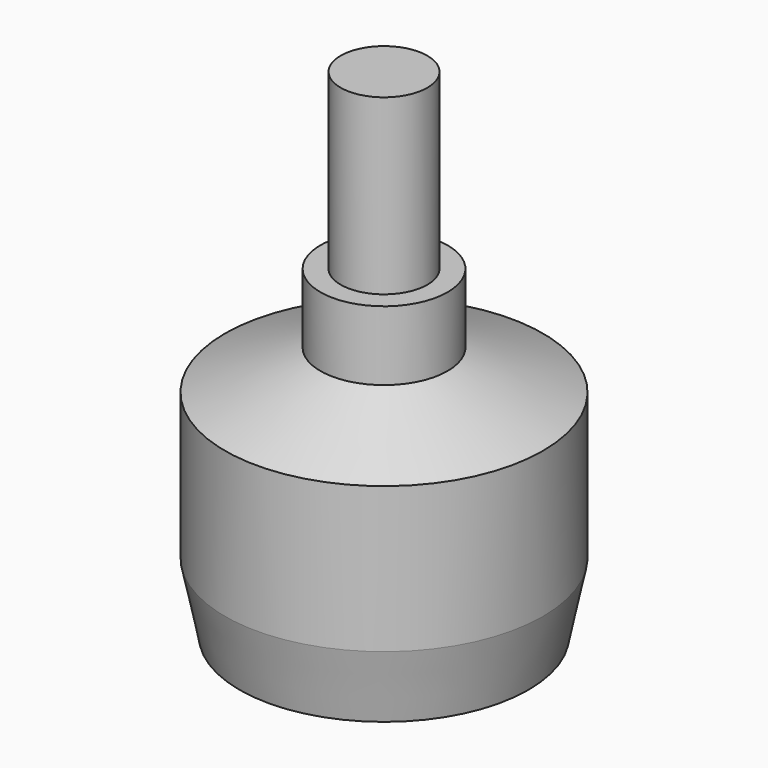
from build123d import *

# Parameters (mm, degrees)
F1_START    = 6
F0_R        = 13.75
F0_R_2      = 12.5
F0_R_3      = 5.5
F0_R_4      = 3.75
F1_DEPTH    = 12.5
F2_DEPTH    = 22
F3_DEPTH    = 28
F4_DEPTH    = 7
F5_SIZE2    = 1.24999
F5_SIZE     = 5.99999
F6_S5_R     = 13.75
F6_T6_DEPTH = 21
F7_DEPTH    = 43


# Not quite as in the source:
# - a fillet or chamfer that OpenCascade refuses, or shapes differently, is made with other operations: its cross-section is extruded or revolved along the edge and cut away or added
# - a fillet or chamfer is up to 0.001 mm smaller than in the source, because OpenCascade refuses the exact size


with BuildPart() as f1:
    # F0 (on Top) → F1 (new body)
    with BuildSketch(Plane.XY.offset(F1_START)):
        Circle(F0_R)
        Circle(F0_R_2, mode=Mode.SUBTRACT)
        Circle(F0_R_2)
        Circle(F0_R_3, mode=Mode.SUBTRACT)
        Circle(F0_R_3)
        Circle(F0_R_4, mode=Mode.SUBTRACT)
        Circle(F0_R_4)
    extrude(amount=F1_DEPTH)

    # F0 (on Top) → F2 (join)
    with BuildSketch(Plane.XY):
        Circle(F0_R_3)
        Circle(F0_R_4, mode=Mode.SUBTRACT)
        Circle(F0_R_4)
    extrude(amount=F2_DEPTH)

    # F0 (on Top) → F3 (join)
    with BuildSketch(Plane.XY):
        Circle(F0_R_3)
        Circle(F0_R_4, mode=Mode.SUBTRACT)
        Circle(F0_R_4)
    extrude(amount=F3_DEPTH)

    # F0 (on Top) → F4 (join)
    with BuildSketch(Plane.XY):
        Circle(F0_R_2)
        Circle(F0_R_3, mode=Mode.SUBTRACT)
    extrude(amount=F4_DEPTH)

    # F5 (size 6 and 1.25 in the source; OpenCascade refuses exactly that, so slightly less here)
    f5_edges = [f1.edges().sort_by_distance(p)[0] for p in [
        (-12.5, 0, 6),
    ]]
    f5_side = f1.faces().sort_by_distance((-12.5, 0, 3))[0]
    chamfer(f5_edges, length=F5_SIZE, length2=F5_SIZE2, reference=f5_side)

    # F6: chamfer of 8.5 x 3.5 on 1 edges, made by hand


with BuildPart() as f6_tool2:
    # F6_s3 → F6_t4 (revolve)
    with BuildSketch(Plane.XZ):
        Polygon((14, 18.5), (5.5, 22), (5.5, 18.5), align=None)
    revolve(axis=Axis((0, 0, 18.5), (0, 0, -1)))

    # F6_s5 → F6_t6 (intersect, symmetric)
    with BuildSketch(Plane.XY.offset(20.2)):
        Circle(F6_S5_R)
    extrude(amount=F6_T6_DEPTH, both=True, mode=Mode.INTERSECT)


with BuildPart() as f1_1:
    add(f1.part)

    # F6_t1: union F6_tool2
    add(f6_tool2.part)

    # F0 (on Top) → F7 (join)
    with BuildSketch(Plane.XY):
        Circle(F0_R_4)
    extrude(amount=F7_DEPTH)


solid = f1_1.part
